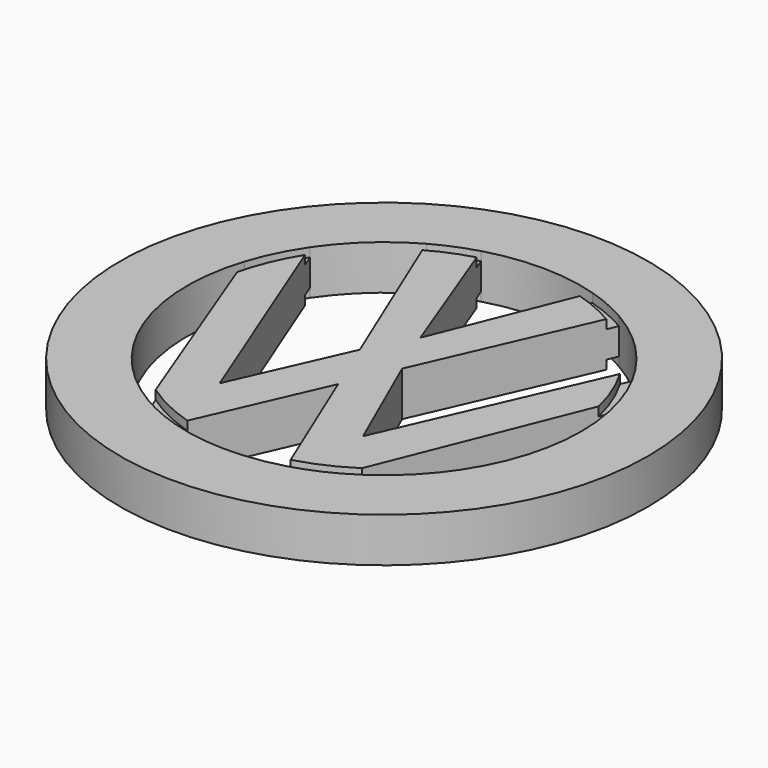
from build123d import *
from build123d import SkipClean  # not in build123d's __all__

# Parameters (mm, degrees)
F0_R     = 118.5
F1_DEPTH = 20
F2_DEPTH = 20
F4_DEPTH = 4
F6_DEPTH = 4


with BuildPart() as f1:
    # F0 (on Top) → F1 (new body)
    with BuildSketch(Plane.XY):
        Circle(F0_R)
        with BuildLine():
            ThreePointArc((84.4585554209, 26.4386538277), (87.4838046576, 13.3728801171), (88.5, 0))
            ThreePointArc((88.5, 0), (76.2236705877, -44.9689008331), (42.8005188217, -77.4620267524))
            ThreePointArc((42.8005188217, -77.4620267524), (33.7736370968, -81.8021481213), (24.3141576643, -85.0944871133))
            ThreePointArc((24.3141576643, -85.0944871133), (-1.1327702213, -88.4927501642), (-26.4843739752, -84.4442297327))
            ThreePointArc((-26.4843739752, -84.4442297327), (-35.8564791301, -80.9108330472), (-44.7693079971, -76.3410706072))
            ThreePointArc((-44.7693079971, -76.3410706072), (-82.6573501675, -31.6229736629), (-84.2920148647, 26.9649073806))
            ThreePointArc((-84.2920148647, 26.9649073806), (-79.5306754268, 38.821664907), (-73.1116226226, 49.869235381))
            ThreePointArc((-73.1116226226, 49.869235381), (-59.6374598942, 65.3882510652), (-42.9470514929, 77.3808811533))
            ThreePointArc((-42.9470514929, 77.3808811533), (-33.9284003129, 81.7380795726), (-24.4751691036, 85.0483162523))
            ThreePointArc((-24.4751691036, 85.0483162523), (0.6651888823, 88.4975000989), (25.7508578518, 84.6707937833))
            ThreePointArc((25.7508578518, 84.6707937833), (35.1532611727, 81.2188292758), (44.1053955412, 76.7265539703))
            ThreePointArc((44.1053955412, 76.7265539703), (60.8748593955, 64.2378509414), (74.2463940977, 48.1635024005))
            ThreePointArc((74.2463940977, 48.1635024005), (80.0924934797, 37.6489374113), (84.4585554209, 26.4386538277))
        make_face(mode=Mode.SUBTRACT)
    extrude(amount=F1_DEPTH)

    # F0 (on Top) → F2 (join)
    with BuildSketch(Plane.XY):
        with BuildLine():
            Line((-84.2920148647, 26.9649073806), (-44.7693079971, -76.3410706072))
            Line((-44.7693079971, -76.3410706072), (-33.3414858158, -50.5729274495))
            Line((-33.3414858158, -50.5729274495), (-73.1116226226, 49.869235381))
            ThreePointArc((-73.1116226226, 49.869235381), (-79.5306754268, 38.821664907), (-84.2920148647, 26.9649073806))
        make_face()
        with BuildLine():
            ThreePointArc((-44.7693079971, -76.3410706072), (-35.8564791301, -80.9108330472), (-26.4843739752, -84.4442297327))
            Line((-26.4843739752, -84.4442297327), (-0.5078915586, -25.1346434059))
            Line((-0.5078915586, -25.1346434059), (-10.9130780509, 0))
            Line((-10.9130780509, 0), (-33.3414858158, -50.5729274495))
            Line((-33.3414858158, -50.5729274495), (-44.7693079971, -76.3410706072))
        make_face()
        with BuildLine():
            Line((9.6563450565, -1.9276264085), (44.1053955412, 76.7265539703))
            ThreePointArc((44.1053955412, 76.7265539703), (35.1532611727, 81.2188292758), (25.7508578518, 84.6707937833))
            Line((25.7508578518, 84.6707937833), (0, 20.3185360879))
            Line((0, 20.3185360879), (-24.4751691036, 85.0483162523))
            ThreePointArc((-24.4751691036, 85.0483162523), (-33.9284003129, 81.7380795726), (-42.9470514929, 77.3808811533))
            Line((-42.9470514929, 77.3808811533), (-10.9130780509, 0))
            Line((-10.9130780509, 0), (-0.5078915586, -25.1346434059))
            Line((-0.5078915586, -25.1346434059), (9.6563450565, -1.9276264085))
        make_face()
        with BuildLine():
            ThreePointArc((24.3141576643, -85.0944871133), (33.7736370968, -81.8021481213), (42.8005188217, -77.4620267524))
            Line((42.8005188217, -77.4620267524), (31.0016963563, -50.5729274495))
            Line((31.0016963563, -50.5729274495), (9.6563450565, -1.9276264085))
            Line((9.6563450565, -1.9276264085), (-0.5078915586, -25.1346434059))
            Line((-0.5078915586, -25.1346434059), (24.3141576643, -85.0944871133))
        make_face()
        with BuildLine():
            Line((42.8005188217, -77.4620267524), (84.4585554209, 26.4386538277))
            ThreePointArc((84.4585554209, 26.4386538277), (80.0924934797, 37.6489374113), (74.2463940977, 48.1635024005))
            Line((74.2463940977, 48.1635024005), (31.0016963563, -50.5729274495))
            Line((31.0016963563, -50.5729274495), (42.8005188217, -77.4620267524))
        make_face()
    extrude(amount=F2_DEPTH)

    # F3 (on face) → F4 (cut)
    with BuildSketch(Plane.XY.offset(20)):
        with BuildLine():
            ThreePointArc((24.3141576643, -85.0944871133), (33.7736370968, -81.8021481213), (42.8005188217, -77.4620267524))
            Line((42.8005188217, -77.4620267524), (45.8884559448, -69.7603011103))
            ThreePointArc((45.8884559448, -69.7603011103), (34.5537158667, -76.0150690311), (22.3883760006, -80.4425920769))
            Line((22.3883760006, -80.4425920769), (24.3141576643, -85.0944871133))
        make_face()
        with BuildLine():
            ThreePointArc((-44.7693079971, -76.3410706072), (-35.8564791301, -80.9108330472), (-26.4843739752, -84.4442297327))
            Line((-26.4843739752, -84.4442297327), (-24.4657542833, -79.8353109053))
            ThreePointArc((-24.4657542833, -79.8353109053), (-36.5644517119, -75.068574457), (-47.7763395541, -68.4811753609))
            Line((-47.7763395541, -68.4811753609), (-44.7693079971, -76.3410706072))
        make_face()
        with BuildLine():
            ThreePointArc((-73.1116226226, 49.869235381), (-79.5306754268, 38.821664907), (-84.2920148647, 26.9649073806))
            Line((-84.2920148647, 26.9649073806), (-81.2849833078, 19.1050121343))
            ThreePointArc((-81.2849833078, 19.1050121343), (-77.0970321509, 32.067080215), (-70.8572793817, 44.1757394803))
            Line((-70.8572793817, 44.1757394803), (-73.1116226226, 49.869235381))
        make_face()
        with BuildLine():
            Line((-22.7005830367, 80.3550466977), (-24.4751691036, 85.0483162523))
            ThreePointArc((-24.4751691036, 85.0483162523), (-33.9284003129, 81.7380795726), (-42.9470514929, 77.3808811533))
            Line((-42.9470514929, 77.3808811533), (-41.0212698292, 72.728986117))
            ThreePointArc((-41.0212698292, 72.728986117), (-32.0882818667, 77.0882102973), (-22.7005830367, 80.3550466977))
        make_face()
        with BuildLine():
            Line((42.0867758493, 72.117635143), (44.1053955412, 76.7265539703))
            ThreePointArc((44.1053955412, 76.7265539703), (35.1532611727, 81.2188292758), (25.7508578518, 84.6707937833))
            Line((25.7508578518, 84.6707937833), (23.8860818979, 80.0106561126))
            ThreePointArc((23.8860818979, 80.0106561126), (33.2216711626, 76.6065960943), (42.0867758493, 72.117635143))
        make_face()
        with BuildLine():
            Line((81.3706182978, 18.7369281856), (84.4585554209, 26.4386538277))
            ThreePointArc((84.4585554209, 26.4386538277), (80.0924934797, 37.6489374113), (74.2463940977, 48.1635024005))
            Line((74.2463940977, 48.1635024005), (71.8122254689, 42.6058009338))
            ThreePointArc((71.8122254689, 42.6058009338), (77.515654404, 31.0414774507), (81.3706182978, 18.7369281856))
        make_face()
    with SkipClean():  # cleaning this boolean's faces spoils the solid; the shape is the same uncleaned
        extrude(amount=-F4_DEPTH, mode=Mode.SUBTRACT)

    # F5 (on face) → F6 (cut)
    with BuildSketch(Plane(origin=(0, 0, 0), x_dir=(1, 0, 0), z_dir=(0, 0, -1))):
        with BuildLine():
            Line((-24.4657542833, 79.8353109053), (-26.4843739752, 84.4442297327))
            ThreePointArc((-26.4843739752, 84.4442297327), (-35.8564791301, 80.9108330472), (-44.7693079971, 76.3410706072))
            Line((-44.7693079971, 76.3410706072), (-47.7763395541, 68.4811753609))
            ThreePointArc((-47.7763395541, 68.4811753609), (-36.5644517119, 75.068574457), (-24.4657542833, 79.8353109053))
        make_face()
        with BuildLine():
            Line((45.8884559448, 69.7603011104), (42.8005188217, 77.4620267524))
            ThreePointArc((42.8005188217, 77.4620267524), (33.7736370968, 81.8021481213), (24.3141576643, 85.0944871133))
            Line((24.3141576643, 85.0944871133), (22.3883760006, 80.4425920769))
            ThreePointArc((22.3883760006, 80.4425920769), (34.5537158667, 76.0150690311), (45.8884559448, 69.7603011103))
        make_face()
        with BuildLine():
            ThreePointArc((74.2463940977, -48.1635024005), (80.0924934797, -37.6489374113), (84.4585554209, -26.4386538277))
            Line((84.4585554209, -26.4386538277), (81.3706182978, -18.7369281856))
            ThreePointArc((81.3706182978, -18.7369281856), (77.515654404, -31.0414774507), (71.8122254689, -42.6058009338))
            Line((71.8122254689, -42.6058009338), (74.2463940977, -48.1635024005))
        make_face()
        with BuildLine():
            ThreePointArc((25.7508578518, -84.6707937833), (35.1532611727, -81.2188292758), (44.1053955412, -76.7265539703))
            Line((44.1053955412, -76.7265539703), (42.0867758493, -72.117635143))
            ThreePointArc((42.0867758493, -72.117635143), (33.2216711626, -76.6065960943), (23.8860818979, -80.0106561126))
            Line((23.8860818979, -80.0106561126), (25.7508578518, -84.6707937833))
        make_face()
        with BuildLine():
            ThreePointArc((-42.9470514929, -77.3808811533), (-33.9284003129, -81.7380795726), (-24.4751691036, -85.0483162523))
            Line((-24.4751691036, -85.0483162523), (-22.7005830367, -80.3550466977))
            ThreePointArc((-22.7005830367, -80.3550466977), (-32.0882818667, -77.0882102973), (-41.0212698292, -72.728986117))
            Line((-41.0212698292, -72.728986117), (-42.9470514929, -77.3808811533))
        make_face()
        with BuildLine():
            Line((-81.2849833078, -19.1050121343), (-84.2920148647, -26.9649073806))
            ThreePointArc((-84.2920148647, -26.9649073806), (-79.5306754268, -38.821664907), (-73.1116226226, -49.869235381))
            Line((-73.1116226226, -49.869235381), (-70.8572793817, -44.1757394803))
            ThreePointArc((-70.8572793817, -44.1757394803), (-77.0970321509, -32.067080215), (-81.2849833078, -19.1050121343))
        make_face()
    extrude(amount=-F6_DEPTH, mode=Mode.SUBTRACT)


solid = f1.part
